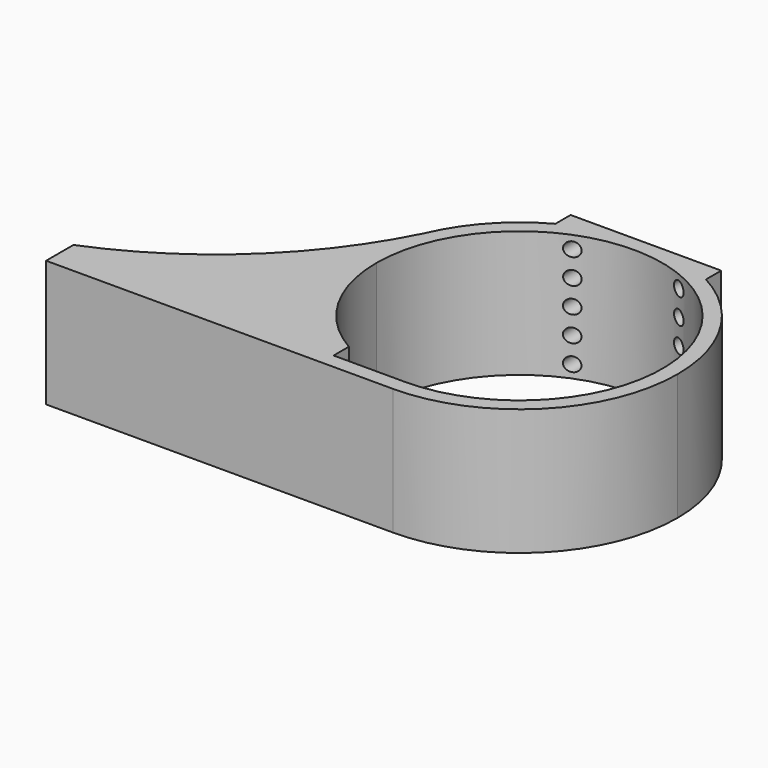
from build123d import *

# Parameters (mm, degrees)
F1_DEPTH = 32.004
F3_DEPTH = 76.54355
F4_R     = 1.778
F5_DEPTH = 44.60469
F7_DEPTH = 32.004


# Not quite as in the source:
# - ends of sketch curves that miss each other by under 0.0002 mm in the source are joined


with BuildPart() as f1:
    # F0 (on Top) → F1 (new body)
    with BuildSketch(Plane.XY):
        with BuildLine():
            Line((-6.8850605494, 65.9121533447), (-6.8850605494, 61.0852363653))
            ThreePointArc((-6.8850605494, 61.0852363653), (-22.2043438922, 46.3803648051), (-27.8400605494, 25.9071533447))
            ThreePointArc((-27.8400605494, 25.9071533447), (-23.8462320221, 8.4831597105), (-12.6621800762, -5.4618466553))
            Line((-12.6621800762, -5.4618466553), (-75.5756720901, -5.4618466553))
            Line((-75.5756720901, -5.4618466553), (-75.5756720901, -14.0978466553))
            Line((-75.5756720901, -14.0978466553), (12.1649394506, -14.0978466553))
            ThreePointArc((12.1649394506, -14.0978466553), (40.452746232, -2.3806534366), (52.1699394506, 25.9071533447))
            ThreePointArc((52.1699394506, 25.9071533447), (46.5342227935, 46.3803648051), (31.2149394506, 61.0852363653))
            Line((31.2149394506, 61.0852363653), (31.2149394506, 65.9121533447))
            Line((31.2149394506, 65.9121533447), (12.1649394506, 65.9121533447))
            Line((12.1649394506, 65.9121533447), (-6.8850605494, 65.9121533447))
        make_face()
        with BuildLine():
            Line((-5.8923298493, -10.2878466553), (-5.8923298493, -5.4618466553))
            ThreePointArc((-5.8923298493, -5.4618466553), (-19.1692254039, 7.7895338028), (-24.0300605494, 25.9071533447))
            ThreePointArc((-24.0300605494, 25.9071533447), (12.1649394506, 62.1021533447), (48.3599394506, 25.9071533447))
            ThreePointArc((48.3599394506, 25.9071533447), (37.7586693957, 0.3134233997), (12.1649394506, -10.2878466553))
            Line((12.1649394506, -10.2878466553), (-5.8923298493, -10.2878466553))
        make_face(mode=Mode.SUBTRACT)
    extrude(amount=F1_DEPTH)

    # F2 (on face) → F3 (cut)
    with BuildSketch(Plane(origin=(-75.5756720901, 0, 0), x_dir=(0, -1, 0), z_dir=(-1, 0, 0))):
        with BuildLine():
            Line((5.4618466553, 28.702), (5.4618466553, 3.302))
            ThreePointArc((5.4618466553, 3.302), (10.2879432961, 16.002), (5.4618466553, 28.702))
        make_face()
    extrude(amount=-F3_DEPTH, mode=Mode.SUBTRACT)

    # F4 (on face) → F5 (cut)
    with BuildSketch(Plane(origin=(0, 65.9121533447, 0), x_dir=(-1, 0, 0), z_dir=(0, 1, 0))):
        with Locations((-25.6732087171, 22.4042255431)):
            Circle(F4_R)
        with Locations((-25.6569720394, 28.7826433778)):
            Circle(F4_R)
        with Locations((-25.6396394506, 16.002)):
            Circle(F4_R)
        with Locations((-25.6375241614, 9.5933126286)):
            Circle(F4_R)
        with Locations((-25.6380084491, 3.1869229861)):
            Circle(F4_R)
        with Locations((1.3113915509, 3.1869229861)):
            Circle(F4_R)
        with Locations((1.3118758386, 9.5933126286)):
            Circle(F4_R)
        with Locations((1.3097605494, 16.002)):
            Circle(F4_R)
        with Locations((1.2761912829, 22.4042255431)):
            Circle(F4_R)
        with Locations((1.2924279606, 28.7826433778)):
            Circle(F4_R)
    extrude(amount=-F5_DEPTH, mode=Mode.SUBTRACT)

    # F6 (on face) → F7 (join)
    with BuildSketch(Plane.XY.offset(32.004)):
        with BuildLine():
            ThreePointArc((-24.5815716288, 41.7215122786), (-45.7821906846, 13.486402418), (-75.5756720901, -5.4618466553))
            Line((-75.5756720901, -5.4618466553), (-12.6621800762, -5.4618466553))
            ThreePointArc((-12.6621800762, -5.4618466553), (-23.9121515851, 16.7934110455), (-24.5815716288, 41.7215122786))
        make_face()
    extrude(amount=-F7_DEPTH)


solid = f1.part
